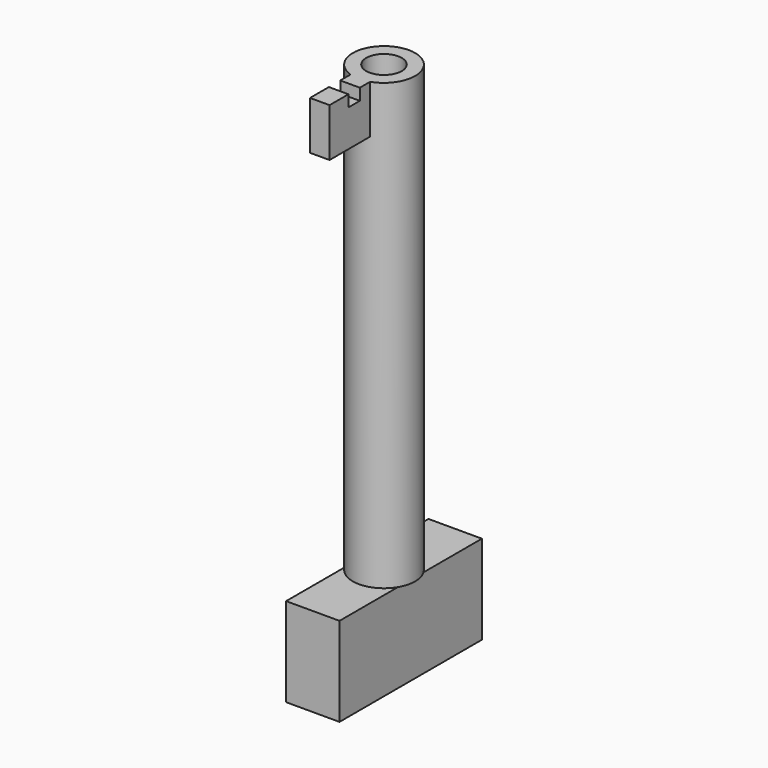
from build123d import *

# Parameters (mm, degrees)
F0_R          = 3.5
F0_R_2        = 2
F1_DEPTH      = 50
F2_W          = 2.2
F2_H          = 5.43
F3_DEPTH      = 9.02
F4_END_RADIUS = 2
F4_REACH      = 14.8797455995
F5_W          = 2.2
F5_H          = 1.6
F6_DEPTH      = 1.3
F7_W          = 6
F7_H          = 20
F8_DEPTH      = 10


with BuildPart() as f1:
    # F0 (on Top) → F1 (new body)
    with BuildSketch(Plane.XY):
        Circle(F0_R)
        Circle(F0_R_2, mode=Mode.SUBTRACT)
    extrude(amount=F1_DEPTH)

    # F2 (on Front) → F3 (join)
    with BuildSketch(Plane.XZ):
        with Locations((0, 47.285)):
            Rectangle(F2_W, F2_H)
    extrude(amount=F3_DEPTH)

    f4_end = (Plane(origin=(0, 0, 25), x_dir=(-1, 0, 0), z_dir=(0, 0, -1)) * Cylinder(F4_END_RADIUS, 133.7931472917, mode=Mode.PRIVATE)).faces().sort_by_distance((-2, 0, 25))[0]
    # F2 (on Front) → F4 (cut, up to the whole of a round face its end follows)
    with BuildSketch(Plane.XZ):
        with Locations((0, 47.285)):
            Rectangle(F2_W, F2_H)
    f4_long = extrude(amount=F4_REACH, mode=Mode.PRIVATE)
    add(split(f4_long, bisect_by=f4_end, keep=Keep.BOTTOM, mode=Mode.PRIVATE), mode=Mode.SUBTRACT)

    # F5 (on face) → F6 (cut)
    with BuildSketch(Plane.XY.offset(50)):
        with Locations((0, -5.57)):
            Rectangle(F5_W, F5_H)
    extrude(amount=-F6_DEPTH, mode=Mode.SUBTRACT)

    # F7 (on face) → F8 (join)
    with BuildSketch(Plane(origin=(0, 0, 0), x_dir=(1, 0, 0), z_dir=(0, 0, -1))):
        Rectangle(F7_W, F7_H)
    extrude(amount=F8_DEPTH)


solid = f1.part
